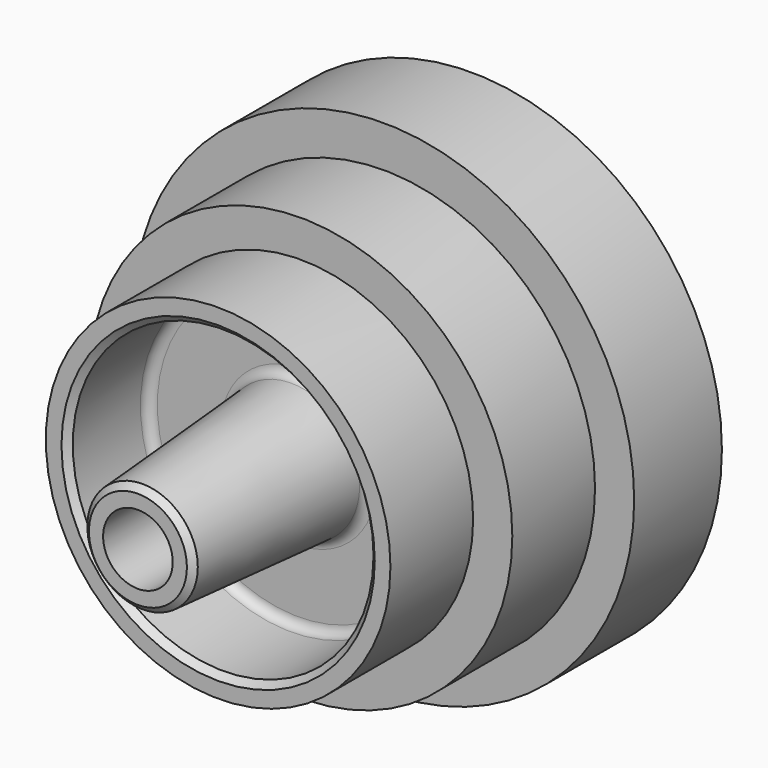
from build123d import *

# Parameters (mm, degrees)
F3_R      = 80
F4_DEPTH  = 35
F5_R      = 67.5
F6_DEPTH  = 33
F7_R      = 55
F8_DEPTH  = 33
F9_R      = 48
F10_DEPTH = 64
F11_R     = 22
F12_R     = 17.5
F14_R     = 74
F15_DEPTH = 27
F16_R     = 61
F17_DEPTH = 60.001
F18_R     = 22
F19_R     = 17.5
F21_R     = 11.11
F22_DEPTH = 133.0010001
F24_R     = 3


# Not quite as in the source:
# - a fillet or chamfer that OpenCascade refuses, or shapes differently, is made with other operations: its cross-section is extruded or revolved along the edge and cut away or added


with BuildPart() as f4:
    # F3 (on Front) → F4 (new body)
    with BuildSketch(Plane.XZ):
        Circle(F3_R)
    extrude(amount=F4_DEPTH)

    # F5 (on face) → F6 (join)
    with BuildSketch(Plane.XZ.offset(35)):
        with Locations((-1.0126e-06, -0.7260435959)):
            Circle(F5_R)
    extrude(amount=F6_DEPTH)

    # F7 (on face) → F8 (join)
    with BuildSketch(Plane.XZ.offset(68)):
        Circle(F7_R)
    extrude(amount=F8_DEPTH)

    # F9 (on offset) → F10 (cut)
    with BuildSketch(Plane.XZ.offset(133)):
        Circle(F9_R)
    extrude(amount=-F10_DEPTH, mode=Mode.SUBTRACT)

    # F11 (on face) → F13 section 0
    with BuildSketch(Plane.XZ.offset(69)):
        Circle(F11_R)
    # F12 (on offset) → F13 section 1
    with BuildSketch(Plane.XZ.offset(133)):
        Circle(F12_R)
    loft()

    # F14 (on Front) → F15 (cut)
    with BuildSketch(Plane.XZ):
        Circle(F14_R)
    extrude(amount=F15_DEPTH, mode=Mode.SUBTRACT)

    # F16 (on offset) → F17 (cut, through all)
    with BuildSketch(Plane.XZ.offset(60)):
        with Locations((0, -3.5063521937)):
            Circle(F16_R)
    extrude(amount=-F17_DEPTH, mode=Mode.SUBTRACT)

    # F18 (on face) → F20 section 0
    with BuildSketch(Plane(origin=(0, -60, 0), x_dir=(-1, 0, 0), z_dir=(0, 1, 0))):
        Circle(F18_R)
    # F19 (on offset) → F20 section 1
    with BuildSketch(Plane.XZ.offset(28)):
        Circle(F19_R)
    loft()

    # F21 (on Front) → F22 (cut, through all)
    with BuildSketch(Plane.XZ):
        Circle(F21_R)
    extrude(amount=F22_DEPTH, mode=Mode.SUBTRACT)

    # F23: chamfer of 2 on 2 edges, made by hand

    # F23_s1 → F23_t2 (revolve, cut)
    with BuildSketch(Plane.XY):
        Polygon((50, -101), (48, -99), (48, -101), align=None)
    revolve(axis=Axis((0, -101, 0), (0, -1, 0)), mode=Mode.SUBTRACT)

    # F23_s3 → F23_t4 (revolve, cut)
    with BuildSketch(Plane.XY):
        Polygon((17.6307616561, -131.1402786693), (15.6356872477, -133), (17.5, -133), align=None)
    revolve(axis=Axis((0, -133, 0), (0, -1, 0)), mode=Mode.SUBTRACT)

    # F24
    f24_edges = [f4.edges().sort_by_distance(p)[0] for p in [
        (-22, -69, 0),
        (-48, -69, 0),
        (-61, -60, -3.506352),
        (22, -60, 0),
    ]]
    fillet(f24_edges, radius=F24_R)


solid = f4.part
